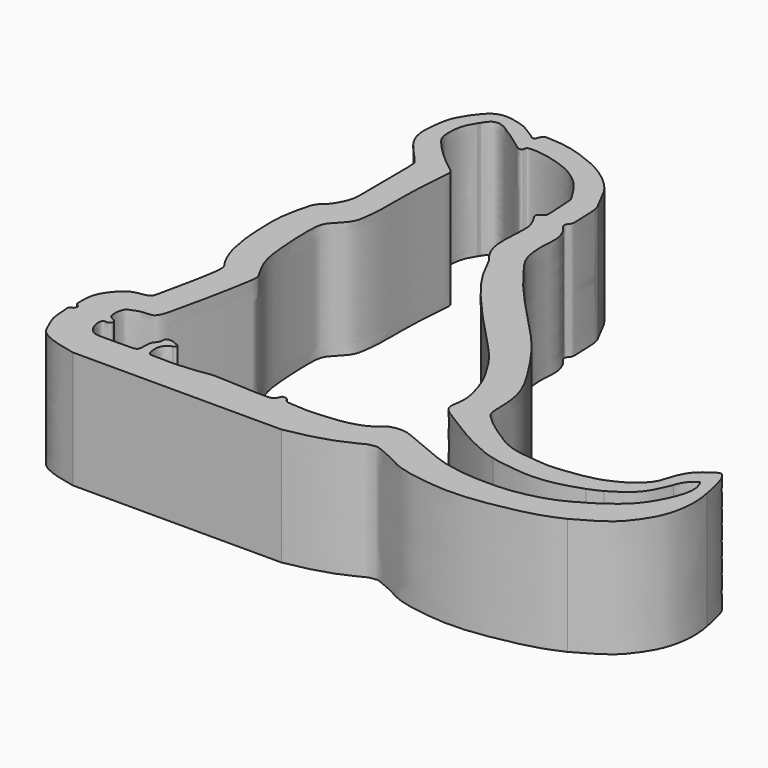
from build123d import *

# Parameters (mm, degrees)
F1_DEPTH = 5.08


with BuildPart() as f1:
    # F0 (on Top) → F1 (new body)
    with BuildSketch(Plane.XY):
        with BuildLine():
            add(Edge.make_bspline(
                [(-11.4531535655, 17.9316624999), (-11.3423634009, 17.8226080387), (-11.0990398713, 17.5830965577), (-10.5216537315, 17.1752428127), (-9.9832375082, 16.8116000023), (-9.3302766014, 16.5049497915), (-8.5351497911, 16.4210907342), (-7.6826916981, 16.3193589), (-6.9889404844, 16.398664447), (-6.4101964363, 16.4684482113), (-5.6925140638, 16.6154358699), (-5.2172506174, 16.8300922836), (-4.737926802, 17.0715715686), (-4.3068785624, 17.4497022766), (-4.1346039941, 17.6858196333), (-4.0643941611, 17.826827243)],
                knots=[0, 0, 0, 0, 0.042419574, 0.0931642308, 0.1423699622, 0.1931044872, 0.2473970709, 0.3037382441, 0.353898392, 0.4004323317, 0.4518808925, 0.4957535606, 0.5399514919, 0.5853730988, 0.6259275813, 0.6259275813, 0.6259275813, 0.6259275813], degree=3))
            add(Edge.make_bspline(
                [(-11.4531535655, 17.9316624999), (-11.5353278284, 18.0013325693), (-11.599494506, 18.1546413097), (-11.6392459174, 18.4329153399), (-11.6321864133, 19.5729774369), (-12.121309762, 20.7408570607), (-13.2308142182, 22.3617998661), (-13.8442255961, 23.2013966392), (-16.3773954957, 25.7550440824), (-17.205806736, 26.9338284954), (-17.893694871, 27.7744469667), (-17.9002010475, 29.021400573), (-17.8184822247, 29.5057983061), (-17.9897855014, 30.0497916449), (-18.1881615527, 30.275766195), (-18.2946934326, 30.4049965252), (-18.2620452332, 30.5813836452), (-18.1277397895, 30.6574477694), (-18.1285761686, 31.0906791932), (-18.1624494507, 31.9344986736), (-18.2120670314, 32.1457449013), (-18.2822644711, 32.2766117752)],
                knots=[0.1821779851, 0.1821779851, 0.1821779851, 0.1821779851, 0.1987968455, 0.2156710174, 0.2494905898, 0.2877760322, 0.3323884407, 0.3678427424, 0.4293232275, 0.4698632522, 0.5029651526, 0.5385501207, 0.5620196375, 0.58602784, 0.6039449868, 0.6168302331, 0.629630365, 0.6412448386, 0.6621791519, 0.6923850095, 0.7125211911, 0.7125211911, 0.7125211911, 0.7125211911], degree=3))
            add(Edge.make_bspline(
                [(-18.2822644711, 32.2766117752), (-18.3764124539, 32.4691395294), (-18.5746716934, 32.8745694176), (-18.9547100724, 33.5767458928), (-19.8713796985, 34.3090133343), (-20.6712786085, 34.6655738311), (-21.5630569798, 34.9977244911), (-22.289607185, 35.0857544204), (-22.739681166, 35.1104890737), (-22.8902895116, 35.0922607106), (-22.9567494288, 34.9547105739), (-22.9959628259, 34.85761112), (-23.0162381196, 34.789313499), (-23.0410310579, 34.7767824349), (-23.0424862006, 34.7761286919)],
                knots=[0, 0, 0, 0, 0.0875488863, 0.1843626926, 0.3004828811, 0.4033844393, 0.5086232519, 0.6027505646, 0.6738982423, 0.7129539346, 0.7530518454, 0.7894959828, 0.8210273533, 0.8229308962, 0.8229308962, 0.8229308962, 0.8229308962], degree=3))
            add(Edge.make_bspline(
                [(-23.0424862006, 34.7761286919), (-23.0449273652, 34.7750319649), (-23.0474912695, 34.7741032154), (-23.0501528602, 34.7733159161)],
                knots=[0.8229308962, 0.8229308962, 0.8229308962, 0.8229308962, 0.8261243023, 0.8261243023, 0.8261243023, 0.8261243023], degree=3))
            add(Edge.make_bspline(
                [(-23.0501528602, 34.7733159161), (-23.0545410802, 34.7718037439), (-23.0658169935, 34.7685198591), (-23.0800204513, 34.7682348796), (-23.0884888755, 34.7688855933)],
                knots=[0.0021581351, 0.0021581351, 0.0021581351, 0.0021581351, 0.005798454, 0.0111263901, 0.0111263901, 0.0111263901, 0.0111263901], degree=3))
            add(Edge.make_bspline(
                [(-23.0884888755, 34.7688855933), (-23.1003779199, 34.7686586533), (-23.1328950749, 34.7691224435), (-23.1675617858, 34.7535809385), (-23.1907266171, 34.8047911582), (-23.2061327949, 34.8275179634)],
                knots=[0.8400573422, 0.8400573422, 0.8400573422, 0.8400573422, 0.8525582929, 0.8747680855, 0.9015857102, 0.9015857102, 0.9015857102, 0.9015857102], degree=3))
            add(Edge.make_bspline(
                [(-23.2061327949, 34.8275179634), (-23.2333559253, 34.8463304823), (-23.2647020116, 34.8687780005), (-23.2981565972, 34.8923575129)],
                knots=[0.0280714161, 0.0280714161, 0.0280714161, 0.0280714161, 0.0354838753, 0.0354838753, 0.0354838753, 0.0354838753], degree=3))
            add(Edge.make_bspline(
                [(-23.2981565972, 34.8923575129), (-23.2988767288, 34.892762275), (-23.3248742022, 34.9074866854), (-23.3553511069, 34.9290724478), (-23.3874430501, 34.9538305609)],
                knots=[0.9407451714, 0.9407451714, 0.9407451714, 0.9407451714, 0.9414461456, 0.9659304091, 0.9659304091, 0.9659304091, 0.9659304091], degree=3))
            add(Edge.make_bspline(
                [(-23.3874430501, 34.9538305609), (-23.3931059977, 34.9575991511), (-23.5183257902, 35.0402229402), (-23.6443291251, 35.1054632176), (-23.7584039569, 35.1838432252)],
                knots=[0.0418291952, 0.0418291952, 0.0418291952, 0.0418291952, 0.0430086944, 0.0678657162, 0.0678657162, 0.0678657162, 0.0678657162], degree=3))
            add(Edge.make_bspline(
                [(-26.1538624763, 34.1210328043), (-26.1307370492, 34.1751880638), (-26.0822982029, 34.2886224609), (-25.9658399245, 34.4784520857), (-25.8367286637, 34.7222051807), (-25.6728345837, 34.9333072266), (-25.4439024159, 35.211302267), (-25.2265629641, 35.3669839468), (-24.9870615601, 35.4455267206), (-24.8071553611, 35.4561515908), (-24.6253811619, 35.4452719932), (-24.4282528156, 35.4124563816), (-24.2023609898, 35.3568568595), (-23.9138114794, 35.2698461332), (-23.8380879164, 35.2283194661), (-23.7584039569, 35.1838432252)],
                knots=[0, 0, 0, 0, 0.0671677149, 0.1421214746, 0.2249641321, 0.3079903593, 0.4027612882, 0.4853187471, 0.5636684732, 0.6308045814, 0.6978681882, 0.7682230286, 0.8464364216, 0.9304502691, 1, 1, 1, 1], degree=3))
            add(Edge.make_bspline(
                [(-25.1203924417, 30.8839287609), (-25.1562608207, 30.9362134154), (-25.2475018018, 31.0692136602), (-25.5941633097, 31.4371340123), (-26.0988037641, 31.9831774136), (-26.3235628346, 32.5710825271), (-26.3308719409, 33.0580330838), (-26.267644153, 33.6751860491), (-26.1899151296, 33.9797626196), (-26.1538624763, 34.1210328043)],
                knots=[0, 0, 0, 0, 0.0919674503, 0.2339442329, 0.409585968, 0.566381973, 0.7063931007, 0.8638178216, 1, 1, 1, 1], degree=3))
            add(Edge.make_bspline(
                [(-25.1203924417, 30.8839287609), (-25.0886757261, 30.8488100619), (-25.0858553072, 30.7298281237), (-25.0605183202, 30.5414498556), (-25.0811840994, 29.4385381855), (-25.025121507, 27.8856571604), (-25.0878508685, 27.3842583921), (-25.2783239246, 27.0108607833), (-25.3896626652, 26.7964370834), (-25.5940210314, 26.5788191515), (-25.8230618275, 26.4054110505), (-25.9629958258, 25.978131493), (-26.1101708802, 25.2629515982), (-26.1930934834, 24.6887465002), (-26.1587460044, 23.5953713197), (-26.0923778546, 22.7066225224), (-25.8549842087, 21.6428561237), (-25.4792186965, 21.0084943162), (-25.2488940087, 20.7558964092), (-25.6031770536, 19.1423379832), (-25.8752014488, 17.9034210742)],
                knots=[0.445949678, 0.445949678, 0.445949678, 0.445949678, 0.4606016519, 0.4767201663, 0.5169581501, 0.5660347046, 0.5932453766, 0.6172063162, 0.6362765888, 0.6569197902, 0.677099802, 0.7025270895, 0.7352531162, 0.7651894637, 0.8048239261, 0.8421337262, 0.8826114218, 0.9145317439, 0.9341388234, 1, 1, 1, 1], degree=3))
            add(Edge.make_bspline(
                [(-25.8752014488, 17.9034210742), (-25.890226418, 17.8385940614), (-25.9181016975, 17.7183228602), (-26.0280658323, 17.6086152498), (-26.3580697207, 17.5628266856), (-26.8372170059, 17.4724464527), (-27.3412522543, 16.8823959482), (-27.5876734804, 16.3942447708), (-27.5859384154, 15.7548281184), (-27.559666492, 15.6041924875), (-27.4454298624, 15.5597037984), (-27.4091925648, 15.5164474494), (-27.40446379, 15.4213679956), (-27.4685753547, 15.3262476594), (-27.5338586836, 15.3167507729), (-27.6002461641, 15.2885968197), (-27.6332812217, 15.1859599479), (-27.5983987717, 14.8301530597), (-27.5615282937, 14.3707910049), (-27.4634080296, 14.0958808888), (-27.3264889208, 13.8151837564), (-27.1982899269, 13.4630176243), (-26.9092353443, 13.1931500637), (-26.4150422105, 13.0016663658), (-26.1029425206, 12.9146269902), (-25.6877393944, 12.8221827022), (-25.4437103868, 12.765155333)],
                knots=[0, 0, 0, 0, 0.0344863373, 0.0639855733, 0.1086241936, 0.1641824578, 0.2327490814, 0.2937225355, 0.3559622593, 0.3853098427, 0.4111499512, 0.4294614236, 0.4532568552, 0.4793434925, 0.499421999, 0.5194489997, 0.5434180278, 0.5910075895, 0.64611278, 0.688915408, 0.7331184434, 0.7813380609, 0.8313225626, 0.8883414874, 0.9343006116, 1, 1, 1, 1], degree=3))
            Line((-25.4437103868, 12.765155333), (-16.4025947478, 12.765155333))
            add(Edge.make_bspline(
                [(-16.4025947478, 12.765155333), (-16.1325477154, 12.8121301717), (-15.6410122013, 12.9046834632), (-14.9844065574, 13.0825012477), (-14.3633058233, 13.2783819833), (-13.5688307679, 13.6611160533), (-13.4493540543, 13.7432549192), (-13.1147097273, 13.8045320217), (-12.93922772, 13.7837422569), (-12.1480315577, 13.437274029), (-11.5088259607, 13.0448039918), (-10.2445374068, 12.8357133347), (-9.1498502359, 12.7336593824), (-7.965074114, 12.8220975242), (-6.8232223523, 13.03483049), (-5.6038998247, 13.3021566911), (-4.9807119282, 13.5887327234), (-4.7370914961, 13.6951681509)],
                knots=[0, 0, 0, 0, 0.0553291926, 0.1059431332, 0.158535845, 0.2156720776, 0.2406225556, 0.27495853, 0.3021246856, 0.3581217371, 0.4143329098, 0.4838231748, 0.550330998, 0.6177137492, 0.6856038145, 0.7557468163, 0.8158364686, 0.8158364686, 0.8158364686, 0.8158364686], degree=3))
            add(Edge.make_bspline(
                [(-4.7370914961, 13.6951681509), (-4.6336168572, 13.7497695407), (-4.4022190396, 13.8718733002), (-3.915698601, 14.1583931236), (-3.3189609958, 14.5578766942), (-2.8415437902, 15.1210480371), (-2.393185713, 15.8326132355), (-2.1726225731, 16.5980120919), (-2.106400575, 17.3823937336), (-2.1753231615, 17.9085416842), (-2.2190036252, 18.1177239865)],
                knots=[0, 0, 0, 0, 0.0743850462, 0.1663454691, 0.2702248812, 0.3756822507, 0.4875855348, 0.5966665154, 0.7059543766, 0.810481295, 0.810481295, 0.810481295, 0.810481295], degree=3))
            add(Edge.make_bspline(
                [(-2.2190036252, 18.1177239865), (-2.2518107461, 18.2748347059), (-2.3191938065, 18.5027389298), (-2.4290399311, 18.6979265504), (-2.5020790265, 18.7794991688), (-2.5303655878, 18.8093540446)],
                knots=[0.810481295, 0.810481295, 0.810481295, 0.810481295, 0.8889884113, 0.9480975652, 0.9842665566, 0.9842665566, 0.9842665566, 0.9842665566], degree=3))
            add(Edge.make_bspline(
                [(-2.5303655878, 18.8093540446), (-2.5426701888, 18.8223408596), (-2.5550807251, 18.8351173916), (-2.5674912613, 18.8478939235)],
                knots=[0.9842665566, 0.9842665566, 0.9842665566, 0.9842665566, 1, 1, 1, 1], degree=3))
            add(Edge.make_bspline(
                [(-4.0643941611, 17.826827243), (-3.9865836201, 17.9830999177), (-3.86768057, 18.3397290309), (-3.6416754276, 18.6704218123), (-3.3503084939, 18.8584432296), (-3.0550237105, 18.9017134543), (-2.7920699812, 18.9152360919), (-2.6246045598, 18.893669034), (-2.5674912613, 18.8478939235)],
                knots=[0.6259275813, 0.6259275813, 0.6259275813, 0.6259275813, 0.6708723716, 0.7091205339, 0.7439142078, 0.7767324746, 0.8080795091, 0.8368777612, 0.8368777612, 0.8368777612, 0.8368777612], degree=3))
        make_face()
        with BuildLine():
            add(Edge.make_bspline(
                [(-18.6367090791, 26.806615293), (-18.8379953623, 27.065709235), (-19.2790347915, 27.6334113281), (-19.1385849927, 29.1576934988), (-19.142782507, 29.5768376419), (-19.2364724588, 29.9460879236), (-19.432292799, 30.245707849), (-19.5036923614, 30.3711508025), (-19.452039249, 30.531044358), (-19.1832908953, 30.5779669697), (-19.2042061287, 31.0575192756), (-19.2501349062, 31.946730439), (-19.3048676283, 32.1518750406), (-19.8206112027, 32.9401597753), (-20.1781911638, 33.2766280139), (-20.6657936013, 33.6375280434), (-21.1987273574, 33.8502544994), (-21.8156732253, 34.0369903903), (-22.3532940037, 34.1202740074), (-22.6789525507, 34.1114092951), (-22.781036981, 34.0935154005), (-22.8442123538, 34.0064923878), (-22.836017646, 33.8992917505), (-22.9169687736, 33.8654371785), (-23.0415440189, 33.8778928228), (-23.145046001, 33.9920059469), (-24.3172951647, 34.8056332509), (-24.4709784088, 34.846264388), (-24.6665006085, 34.9235282636), (-24.8730036275, 34.8890028633), (-25.0225147118, 34.7975179285), (-25.1513236902, 34.5965507599), (-25.1965038478, 34.5278270543)],
                knots=[0, 0, 0, 0, 0.0530449929, 0.1162271616, 0.1503362798, 0.1818999441, 0.2130503431, 0.2322815435, 0.2514640261, 0.275217638, 0.3099088569, 0.3591170068, 0.3848334384, 0.4340298475, 0.4724784579, 0.512097197, 0.5519606878, 0.5941304956, 0.6332780537, 0.6623280229, 0.6782450968, 0.6944721334, 0.7106995421, 0.7248499144, 0.7417640264, 0.7633659926, 0.8252786224, 0.8481238707, 0.8706340609, 0.8940154935, 0.9161281592, 0.9453600325, 0.9453600325, 0.9453600325, 0.9453600325], degree=3))
            add(Edge.make_bspline(
                [(-18.6367090791, 26.806615293), (-18.4004431072, 26.3177446993), (-17.8214250743, 25.1196658343), (-14.9958562057, 22.1558553104), (-14.2006384351, 21.3463203299), (-13.4069219143, 20.1028170279), (-13.057819762, 19.1966099457), (-12.8449499507, 18.2061038352), (-13.1501738463, 17.4728388827), (-12.0668415899, 16.9062569537), (-11.2465699819, 16.3394149694), (-10.3042035411, 15.8914402394), (-9.8099199153, 15.6800453052), (-9.4957305118, 15.6079921871)],
                knots=[0, 0, 0, 0, 0.070520737, 0.1729047088, 0.2297494243, 0.2895443737, 0.3410861891, 0.3916345783, 0.432452015, 0.4846611235, 0.5378002653, 0.5889842833, 0.636687273, 0.636687273, 0.636687273, 0.636687273], degree=3))
            add(Edge.make_bspline(
                [(-9.4957305118, 15.6079921871), (-9.1133312834, 15.5202964964), (-8.2008881683, 15.4402897436), (-7.3081707518, 15.4279642007), (-6.2775050816, 15.7326586203), (-5.5702812914, 15.970748713), (-5.1639379173, 16.0504758378), (-5.0442288589, 16.0616629529)],
                knots=[0.636687273, 0.636687273, 0.636687273, 0.636687273, 0.6947464763, 0.7437941737, 0.7961098113, 0.8448976449, 0.8661305735, 0.8661305735, 0.8661305735, 0.8661305735], degree=3))
            add(Edge.make_bspline(
                [(-5.0442288589, 16.0616629529), (-4.9399228548, 16.1184542498), (-4.6922932366, 16.2700279948), (-4.3072979632, 16.5467521861), (-3.9111782293, 16.9402090766), (-3.6467479793, 17.4860351741), (-3.5418440062, 17.7515041171), (-3.4855501726, 17.880808562)],
                knots=[0.1116059668, 0.1116059668, 0.1116059668, 0.1116059668, 0.174466562, 0.2640043057, 0.3569942582, 0.452966765, 0.5340334981, 0.5340334981, 0.5340334981, 0.5340334981], degree=3))
            add(Edge.make_bspline(
                [(-3.4855501726, 17.880808562), (-3.4648551188, 17.9392815903), (-3.4254729985, 18.0505541605), (-3.3592609609, 18.1784369474), (-3.2239072693, 18.3745123065), (-3.075018802, 18.5162428051), (-2.960889175, 18.580902775), (-2.9049660079, 18.6125859618)],
                knots=[0, 0, 0, 0, 0.1933263651, 0.3678947746, 0.5897403457, 0.798974028, 1, 1, 1, 1], degree=3))
            add(Edge.make_bspline(
                [(-2.7946273377, 18.3692199386), (-2.7964008531, 18.3746177266), (-2.8185376651, 18.4405657555), (-2.8607845108, 18.5367806837), (-2.8920297064, 18.5903902465), (-2.9049660079, 18.6125859618)],
                knots=[0.7742104558, 0.7742104558, 0.7742104558, 0.7742104558, 0.7853442377, 0.9111270835, 1, 1, 1, 1], degree=3))
            add(Edge.make_bspline(
                [(-2.7946273377, 18.3692199386), (-2.7819962135, 18.3572528177), (-2.7467831192, 18.3156041133), (-2.6954959966, 18.2431388933), (-2.7118146433, 18.0844860008), (-2.7163067479, 18.0028985872), (-2.7269718703, 17.9558321834)],
                knots=[0.7904142153, 0.7904142153, 0.7904142153, 0.7904142153, 0.8091254065, 0.8492766078, 0.8974005007, 0.94294828, 0.94294828, 0.94294828, 0.94294828], degree=3))
            add(Edge.make_bspline(
                [(-2.7589141579, 17.8106968769), (-2.7480705925, 17.8589856053), (-2.7375212314, 17.9074088943), (-2.7269718703, 17.9558321834)],
                knots=[0.9678475586, 0.9678475586, 0.9678475586, 0.9678475586, 1, 1, 1, 1], degree=3))
            add(Edge.make_bspline(
                [(-2.8583404767, 17.4271704529), (-2.8514740504, 17.4479914895), (-2.8244370396, 17.5313499213), (-2.7886322661, 17.653954814), (-2.7657065006, 17.7682841548), (-2.7589141579, 17.8106968769)],
                knots=[0.0876086045, 0.0876086045, 0.0876086045, 0.0876086045, 0.1340096964, 0.2726867204, 0.3537768689, 0.3537768689, 0.3537768689, 0.3537768689], degree=3))
            add(Edge.make_bspline(
                [(-2.8978604823, 17.3097904772), (-2.8837879349, 17.3485058616), (-2.8706743906, 17.3876598669), (-2.8583404767, 17.4271704529)],
                knots=[0.8542372602, 0.8542372602, 0.8542372602, 0.8542372602, 0.8815008623, 0.8815008623, 0.8815008623, 0.8815008623], degree=3))
            add(Edge.make_bspline(
                [(-4.1314834672, 15.5965547193), (-4.0315274216, 15.6733263507), (-3.7778639874, 15.8777413762), (-3.4320979017, 16.2764907518), (-3.160297974, 16.7462504522), (-2.970488838, 17.1099805481), (-2.8978604823, 17.3097904772)],
                knots=[0.3513635715, 0.3513635715, 0.3513635715, 0.3513635715, 0.4468641765, 0.5821895305, 0.71352993, 0.8542372602, 0.8542372602, 0.8542372602, 0.8542372602], degree=3))
            add(Edge.make_bspline(
                [(-5.1270611584, 14.938313514), (-5.0515530743, 14.9774552199), (-4.8843674391, 15.0641205227), (-4.5469469405, 15.2867318902), (-4.3174529957, 15.4558821713), (-4.1670458139, 15.5692409199), (-4.1314834672, 15.5965547193)],
                knots=[0, 0, 0, 0, 0.092613947, 0.2050604481, 0.3173863808, 0.3513635715, 0.3513635715, 0.3513635715, 0.3513635715], degree=3))
            add(Edge.make_bspline(
                [(-5.1270611584, 14.938313514), (-5.2771142269, 14.8341591333), (-5.6563184579, 14.6364611177), (-6.2827280989, 14.3709318177), (-7.113865798, 14.1755257038), (-7.8061594564, 14.0723005413), (-8.7575945258, 14.062762844), (-9.4755779778, 14.0903441294), (-10.5171680112, 14.2640694268), (-11.0849865282, 14.495208914), (-11.6394734923, 14.7117769501), (-12.3199132485, 14.9929642703), (-12.7929010289, 15.2160549407), (-13.1693051019, 15.3094794414), (-13.6631097568, 15.2406991201), (-13.8878987376, 15.0699376691), (-14.1270175817, 14.8596805039), (-14.4365379063, 14.6998032363), (-14.946365692, 14.5441603648), (-15.4653725357, 14.4701314227), (-16.0228531057, 14.4259051639), (-16.599280406, 14.3831817298), (-17.1563207893, 14.4291134823), (-17.5765573618, 14.4432909445), (-17.6426388891, 14.6781332324), (-17.9252680634, 14.7019285451), (-17.9369295949, 14.4385445784), (-18.1966937306, 14.3022551156), (-19.2514603507, 14.3796871572), (-20.1516024839, 14.4031902832), (-20.7000563565, 14.4503697732), (-21.2012371276, 14.346136563), (-21.6956016992, 14.2977665359), (-22.2745615473, 14.2463720239), (-22.9643071169, 14.2929417537), (-23.4041762898, 14.2443440285), (-23.4357489045, 14.6405144544), (-23.4448194595, 14.9162666216), (-23.2529802358, 15.1376544408), (-23.1260398226, 15.2011345711), (-23.0670906603, 15.2306137607)],
                knots=[0.2264805435, 0.2264805435, 0.2264805435, 0.2264805435, 0.2486079389, 0.2725642119, 0.2988704638, 0.3232808251, 0.3508193168, 0.3758397165, 0.4050386993, 0.427596275, 0.4496366082, 0.4744321143, 0.4951166283, 0.5129757033, 0.5327762454, 0.5479843164, 0.5638359997, 0.5807872712, 0.6016612368, 0.6226275802, 0.6440520809, 0.6659820881, 0.6879120602, 0.7054182805, 0.7182618618, 0.7311197199, 0.7440164781, 0.7580595368, 0.787518082, 0.8155871711, 0.8365634894, 0.8567932415, 0.8769411061, 0.899021601, 0.9233900622, 0.9405536451, 0.956742594, 0.9720531433, 0.9869513902, 1, 1, 1, 1], degree=3))
            add(Edge.make_bspline(
                [(-25.2310526286, 34.4719983222), (-25.3038391294, 34.3540012216), (-25.4531529498, 34.1042935473), (-25.5721470358, 33.7092541942), (-25.587188472, 33.1298241951), (-25.4997983265, 32.7713027421), (-25.0413920552, 32.246510563), (-24.405800543, 31.6505354237), (-23.897365776, 31.2578208694), (-23.7384603201, 31.1382864161), (-23.6760367082, 30.9234858301), (-23.8646136174, 29.371515056), (-23.8160584786, 27.8408048298), (-23.8551271681, 27.1541425133), (-23.9417054048, 26.339591915), (-24.1841815052, 26.0016383593), (-24.5166982086, 25.6736562258), (-24.7714149026, 25.3473157244), (-24.8024256704, 24.6413497116), (-24.7578308739, 23.6496523325), (-24.6946622518, 22.7425708957), (-24.5195394508, 21.8598876019), (-24.0198688435, 21.0761443867), (-23.9591596225, 20.7748494681), (-24.7186554159, 17.060654472), (-24.8645659656, 16.776896027), (-25.0058611967, 16.5379639168), (-25.4743029949, 16.5886627468), (-25.828810169, 16.422282137), (-26.117255434, 16.3440434258), (-26.1701546323, 15.6477142433), (-25.960334184, 15.551537143), (-25.7824829921, 15.4608173801), (-25.7700435102, 15.2730663669), (-25.9120797072, 15.1993096117), (-26.120103391, 15.2497938765), (-26.1587468696, 14.9656310604), (-26.1025293294, 14.7432897715), (-25.9857633015, 14.511549356), (-25.8184734838, 14.331032355), (-25.6147179493, 14.2801439987), (-25.3514809746, 14.2616198502), (-24.4496681404, 14.2701286396), (-24.0407142438, 14.2676187035), (-23.8240741539, 14.3523693205), (-23.8551603339, 14.7361797958), (-23.8173415435, 15.0196417279), (-23.5949082397, 15.2256291566), (-23.6362962994, 15.4703033213), (-23.5144593574, 15.5291150345), (-23.3262235385, 15.5282810576), (-23.1721817841, 15.4584836678), (-22.9132569839, 15.3623304285), (-23.0186889838, 15.2720566209), (-23.0670906603, 15.2306137607)],
                knots=[0.0027278011, 0.0027278011, 0.0027278011, 0.0027278011, 0.0200249886, 0.0393548678, 0.0612294478, 0.0786838853, 0.1025489241, 0.1307470779, 0.1538969322, 0.1658959497, 0.1780571677, 0.2142283318, 0.2513672974, 0.2758186495, 0.3014641695, 0.3202193243, 0.3398196416, 0.3581136586, 0.3821190631, 0.4115331974, 0.439462177, 0.467632387, 0.4942257926, 0.5124318159, 0.5686189168, 0.5863858262, 0.5995567566, 0.6189060586, 0.6372612295, 0.6522652849, 0.6748270314, 0.6879979824, 0.7005384814, 0.7118123465, 0.7226500232, 0.7346799252, 0.7485649543, 0.7629617211, 0.7777715626, 0.7920285271, 0.8046940387, 0.8198234075, 0.84771286, 0.866790111, 0.878951312, 0.8961848444, 0.9120081261, 0.9274768414, 0.9408689641, 0.9504318938, 0.9627680851, 0.9755932763, 0.9887953719, 1, 1, 1, 1], degree=3))
            add(Edge.make_bspline(
                [(-25.1965038478, 34.5278270543), (-25.2109680444, 34.5058255111), (-25.2225466217, 34.4885071169), (-25.2310526286, 34.4719983222)],
                knots=[0.9453600325, 0.9453600325, 0.9453600325, 0.9453600325, 0.9547184674, 0.9547184674, 0.9547184674, 0.9547184674], degree=3))
        make_face(mode=Mode.SUBTRACT)
        with BuildLine():
            add(Edge.make_bspline(
                [(-4.0643941611, 17.826827243), (-4.0329021527, 17.9274360865), (-3.9633756818, 18.1495552272), (-3.8023122301, 18.6095361712), (-3.555300918, 19.0266262674), (-3.1821771361, 19.322271683), (-2.9551182407, 19.4661996221), (-2.846354153, 19.5351429284)],
                knots=[0, 0, 0, 0, 0.1756674888, 0.38782984, 0.6003192445, 0.8085478544, 1, 1, 1, 1], degree=3))
            add(Edge.make_bspline(
                [(-4.0643941611, 17.826827243), (-3.9865836201, 17.9830999177), (-3.86768057, 18.3397290309), (-3.6416754276, 18.6704218123), (-3.3503084939, 18.8584432296), (-3.0550237105, 18.9017134543), (-2.7920699812, 18.9152360919), (-2.6246045598, 18.893669034), (-2.5674912613, 18.8478939235)],
                knots=[0.6259275813, 0.6259275813, 0.6259275813, 0.6259275813, 0.6708723716, 0.7091205339, 0.7439142078, 0.7767324746, 0.8080795091, 0.8368777612, 0.8368777612, 0.8368777612, 0.8368777612], degree=3))
            add(Edge.make_bspline(
                [(-2.5674912613, 18.8478939235), (-2.5538474608, 18.8369587037), (-2.5415202907, 18.824000489), (-2.5303655878, 18.8093540446)],
                knots=[0.8368777612, 0.8368777612, 0.8368777612, 0.8368777612, 0.843757378, 0.843757378, 0.843757378, 0.843757378], degree=3))
            add(Edge.make_bspline(
                [(-2.2190036252, 18.1177239865), (-2.2518107461, 18.2748347059), (-2.3191938065, 18.5027389298), (-2.4290399311, 18.6979265504), (-2.5020790265, 18.7794991688), (-2.5303655878, 18.8093540446)],
                knots=[0.810481295, 0.810481295, 0.810481295, 0.810481295, 0.8889884113, 0.9480975652, 0.9842665566, 0.9842665566, 0.9842665566, 0.9842665566], degree=3))
            add(Edge.make_bspline(
                [(-2.2190036252, 18.1177239865), (-2.2295599779, 18.1909128286), (-2.2525944027, 18.350614094), (-2.3311223768, 18.6665866168), (-2.411011017, 18.9856929483), (-2.5034334632, 19.2962170954), (-2.6620392862, 19.4790050752), (-2.699362075, 19.5283454236), (-2.7892871387, 19.5677127173), (-2.8284091094, 19.5453846817), (-2.846354153, 19.5351429284)],
                knots=[0, 0, 0, 0, 0.1385698593, 0.3023655142, 0.469346878, 0.6353465435, 0.772083198, 0.8437606813, 0.9283338407, 1, 1, 1, 1], degree=3))
        make_face()
        with BuildLine():
            add(Edge.make_bspline(
                [(-9.4957305118, 15.6079921871), (-9.1133312834, 15.5202964964), (-8.2008881683, 15.4402897436), (-7.3081707518, 15.4279642007), (-6.2775050816, 15.7326586203), (-5.5702812914, 15.970748713), (-5.1639379173, 16.0504758378), (-5.0442288589, 16.0616629529)],
                knots=[0.636687273, 0.636687273, 0.636687273, 0.636687273, 0.6947464763, 0.7437941737, 0.7961098113, 0.8448976449, 0.8661305735, 0.8661305735, 0.8661305735, 0.8661305735], degree=3))
            add(Edge.make_bspline(
                [(-9.4957305118, 15.6079921871), (-9.2948678262, 15.5463206649), (-8.7000059095, 15.4649529633), (-7.7290203732, 15.3419949223), (-6.8886297907, 15.4400960431), (-6.2129135882, 15.5896585333), (-5.8190504445, 15.747745542), (-5.6177424267, 15.8075205982)],
                knots=[0, 0, 0, 0, 0.0254322528, 0.0542807701, 0.0806860867, 0.1044391847, 0.1272162238, 0.1272162238, 0.1272162238, 0.1272162238], degree=3))
            add(Edge.make_bspline(
                [(-5.6177424267, 15.8075205982), (-5.466753069, 15.8664520418), (-5.2723213776, 15.9423391137), (-5.0856063663, 16.039134218), (-5.0442288589, 16.0616629529)],
                knots=[0, 0, 0, 0, 0.0866695811, 0.1116059668, 0.1116059668, 0.1116059668, 0.1116059668], degree=3))
        make_face()
        with BuildLine():
            add(Edge.make_bspline(
                [(-2.7946273377, 18.3692199386), (-2.7819962135, 18.3572528177), (-2.7467831192, 18.3156041133), (-2.6954959966, 18.2431388933), (-2.7118146433, 18.0844860008), (-2.7163067479, 18.0028985872), (-2.7269718703, 17.9558321834)],
                knots=[0.7904142153, 0.7904142153, 0.7904142153, 0.7904142153, 0.8091254065, 0.8492766078, 0.8974005007, 0.94294828, 0.94294828, 0.94294828, 0.94294828], degree=3))
            add(Edge.make_bspline(
                [(-2.7498320277, 17.8763530796), (-2.7482850512, 17.8897743927), (-2.7401795828, 17.9706760352), (-2.7408634662, 18.0956768484), (-2.745224744, 18.1928070831), (-2.7747005451, 18.308571691), (-2.7946273377, 18.3692199386)],
                knots=[0.3956408743, 0.3956408743, 0.3956408743, 0.3956408743, 0.4214109088, 0.5516550538, 0.64911396, 0.7742104558, 0.7742104558, 0.7742104558, 0.7742104558], degree=3))
            add(Edge.make_bspline(
                [(-2.7269718703, 17.9558321834), (-2.7325770316, 17.931095966), (-2.7405247135, 17.9043172658), (-2.7498320277, 17.8763530796)],
                knots=[0.94294828, 0.94294828, 0.94294828, 0.94294828, 0.9668863692, 0.9668863692, 0.9668863692, 0.9668863692], degree=3))
        make_face()
        with BuildLine():
            add(Edge.make_bspline(
                [(-23.0884888755, 34.7688855933), (-23.1003779199, 34.7686586533), (-23.1328950749, 34.7691224435), (-23.1675617858, 34.7535809385), (-23.1907266171, 34.8047911582), (-23.2061327949, 34.8275179634)],
                knots=[0.8400573422, 0.8400573422, 0.8400573422, 0.8400573422, 0.8525582929, 0.8747680855, 0.9015857102, 0.9015857102, 0.9015857102, 0.9015857102], degree=3))
            add(Edge.make_bspline(
                [(-23.0884888755, 34.7688855933), (-23.0908912433, 34.7690701912), (-23.1071818944, 34.7707677433), (-23.1325886424, 34.7781756239), (-23.1815038199, 34.8104981332), (-23.2061327949, 34.8275179634)],
                knots=[0.0111263901, 0.0111263901, 0.0111263901, 0.0111263901, 0.0126378475, 0.0213653073, 0.0280714161, 0.0280714161, 0.0280714161, 0.0280714161], degree=3))
        make_face()
        with BuildLine():
            add(Edge.make_bspline(
                [(-2.7589141579, 17.8106968769), (-2.7480705925, 17.8589856053), (-2.7375212314, 17.9074088943), (-2.7269718703, 17.9558321834)],
                knots=[0.9678475586, 0.9678475586, 0.9678475586, 0.9678475586, 1, 1, 1, 1], degree=3))
            add(Edge.make_bspline(
                [(-2.7269718703, 17.9558321834), (-2.7325770316, 17.931095966), (-2.7405247135, 17.9043172658), (-2.7498320277, 17.8763530796)],
                knots=[0.94294828, 0.94294828, 0.94294828, 0.94294828, 0.9668863692, 0.9668863692, 0.9668863692, 0.9668863692], degree=3))
            add(Edge.make_bspline(
                [(-2.7589141579, 17.8106968769), (-2.7554075091, 17.8325930808), (-2.7523451261, 17.854549852), (-2.7498320277, 17.8763530796)],
                knots=[0.3537768689, 0.3537768689, 0.3537768689, 0.3537768689, 0.3956408743, 0.3956408743, 0.3956408743, 0.3956408743], degree=3))
        make_face()
        with BuildLine():
            add(Edge.make_bspline(
                [(-23.2981565972, 34.8923575129), (-23.2988767288, 34.892762275), (-23.3248742022, 34.9074866854), (-23.3553511069, 34.9290724478), (-23.3874430501, 34.9538305609)],
                knots=[0.9407451714, 0.9407451714, 0.9407451714, 0.9407451714, 0.9414461456, 0.9659304091, 0.9659304091, 0.9659304091, 0.9659304091], degree=3))
            add(Edge.make_bspline(
                [(-23.2981565972, 34.8923575129), (-23.3267948721, 34.9125423858), (-23.3569782443, 34.9335567781), (-23.3874430501, 34.9538305609)],
                knots=[0.0354838753, 0.0354838753, 0.0354838753, 0.0354838753, 0.0418291952, 0.0418291952, 0.0418291952, 0.0418291952], degree=3))
        make_face()
        with BuildLine():
            add(Edge.make_bspline(
                [(-2.5674912613, 18.8478939235), (-2.5538474608, 18.8369587037), (-2.5415202907, 18.824000489), (-2.5303655878, 18.8093540446)],
                knots=[0.8368777612, 0.8368777612, 0.8368777612, 0.8368777612, 0.843757378, 0.843757378, 0.843757378, 0.843757378], degree=3))
            add(Edge.make_bspline(
                [(-2.5303655878, 18.8093540446), (-2.5426701888, 18.8223408596), (-2.5550807251, 18.8351173916), (-2.5674912613, 18.8478939235)],
                knots=[0.9842665566, 0.9842665566, 0.9842665566, 0.9842665566, 1, 1, 1, 1], degree=3))
        make_face()
        with BuildLine():
            add(Edge.make_bspline(
                [(-2.8978604823, 17.3097904772), (-2.8845826334, 17.3488246564), (-2.8713047844, 17.3878588357), (-2.8583404767, 17.4271704529)],
                knots=[0, 0, 0, 0, 0.0876086045, 0.0876086045, 0.0876086045, 0.0876086045], degree=3))
            add(Edge.make_bspline(
                [(-2.8978604823, 17.3097904772), (-2.8837879349, 17.3485058616), (-2.8706743906, 17.3876598669), (-2.8583404767, 17.4271704529)],
                knots=[0.8542372602, 0.8542372602, 0.8542372602, 0.8542372602, 0.8815008623, 0.8815008623, 0.8815008623, 0.8815008623], degree=3))
        make_face()
        with BuildLine():
            add(Edge.make_bspline(
                [(-25.1965038478, 34.5278270543), (-25.2080389497, 34.5092168777), (-25.2195740516, 34.4906067012), (-25.2310526286, 34.4719983222)],
                knots=[0, 0, 0, 0, 0.0027278011, 0.0027278011, 0.0027278011, 0.0027278011], degree=3))
            add(Edge.make_bspline(
                [(-25.1965038478, 34.5278270543), (-25.2109680444, 34.5058255111), (-25.2225466217, 34.4885071169), (-25.2310526286, 34.4719983222)],
                knots=[0.9453600325, 0.9453600325, 0.9453600325, 0.9453600325, 0.9547184674, 0.9547184674, 0.9547184674, 0.9547184674], degree=3))
        make_face()
    extrude(amount=F1_DEPTH)


solid = f1.part
